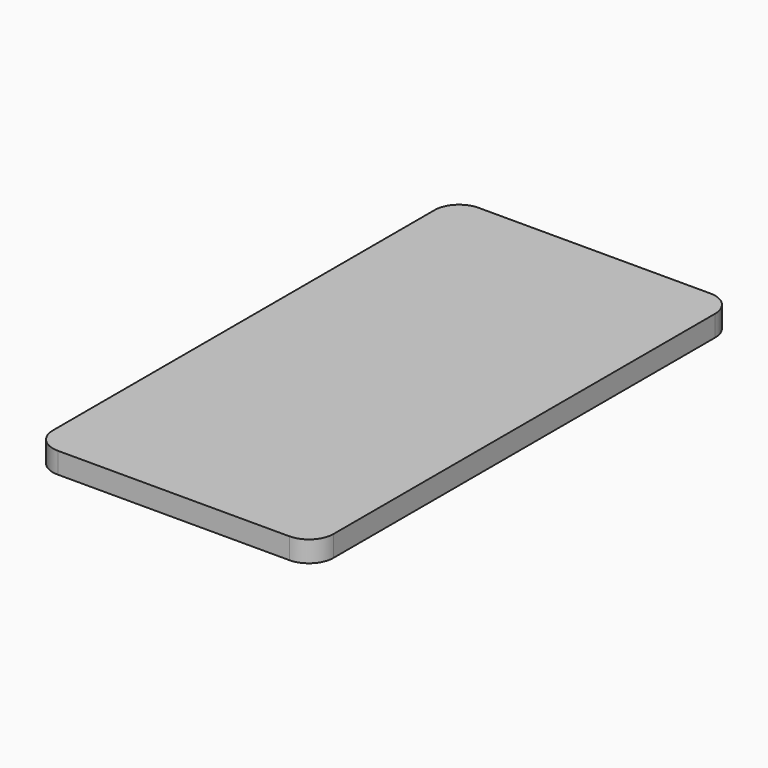
from build123d import *

# Parameters (mm, degrees)
F0_TEXT_SIZE = 202.7059043581
F1_DEPTH     = 152.4
F2_R         = 43.5227402162
F2_R_2       = 31.6103
F2_R_3       = 31.3528753957
F2_R_4       = 28.9308805731
F3_DEPTH     = 152.4
F5_DEPTH     = 154.4


# Not quite as in the source:
# - a feature names something its author has since deleted; it is built from what else it names
# - Text() gives the source's letters only with a copy of the font that has no kerning and outlines rounded to 1/6400 em; it was checked with that copy


with BuildPart() as f1:
    # F0 (on Top) → F1 (new body)
    with BuildSketch(Plane.XY):
        with BuildLine():
            ThreePointArc((0, -177.8), (-52.076414305, -52.076414305), (-177.8, 0))
            Line((-177.8, 0), (-1854.2, 0))
            ThreePointArc((-1854.2, 0), (-1979.923585695, -52.076414305), (-2032, -177.8))
            Line((-2032, -177.8), (-2032, -3632.2))
            ThreePointArc((-2032, -3632.2), (-1979.923585695, -3757.923585695), (-1854.2, -3810))
            Line((-1854.2, -3810), (-177.8, -3810))
            ThreePointArc((-177.8, -3810), (-52.076414305, -3757.923585695), (0, -3632.2))
            Line((0, -3632.2), (0, -177.8))
        make_face()
        with BuildLine():
            add(Edge.make_bspline(
                [(-1427.8888958164, -1437.0154963626), (-1420.3666063969, -1446.754881611), (-1420.3666063969, -1460.9126221185)],
                knots=[0, 0, 0, 1, 1, 1], degree=2))
            add(Edge.make_bspline(
                [(-1420.3666063969, -1460.9126221185), (-1420.3666063969, -1480.5180838057), (-1434.4768377081, -1491.8094361344)],
                knots=[0, 0, 0, 1, 1, 1], degree=2))
            add(Edge.make_bspline(
                [(-1434.4768377081, -1491.8094361344), (-1448.5870690193, -1503.1007884631), (-1473.7035974811, -1503.1007884631)],
                knots=[0, 0, 0, 1, 1, 1], degree=2))
            add(Edge.make_bspline(
                [(-1473.7035974811, -1503.1007884631), (-1496.8880852921, -1503.1007884631), (-1514.6881975185, -1494.3590963376)],
                knots=[0, 0, 0, 1, 1, 1], degree=2))
            Line((-1514.6881975185, -1494.3590963376), (-1514.6881975185, -1465.8535785372))
            add(Edge.make_bspline(
                [(-1514.6881975185, -1465.8535785372), (-1500.0553650477, -1472.4098476313), (-1489.904233431, -1475.070362626)],
                knots=[0, 0, 0, 1, 1, 1], degree=2))
            add(Edge.make_bspline(
                [(-1489.904233431, -1475.070362626), (-1479.7531018143, -1477.7308776207), (-1471.3281376644, -1477.7308776207)],
                knots=[0, 0, 0, 1, 1, 1], degree=2))
            add(Edge.make_bspline(
                [(-1471.3281376644, -1477.7308776207), (-1461.2561880416, -1477.7308776207), (-1455.8559760584, -1473.8826327177)],
                knots=[0, 0, 0, 1, 1, 1], degree=2))
            add(Edge.make_bspline(
                [(-1455.8559760584, -1473.8826327177), (-1450.4557640751, -1470.0343878146), (-1450.4557640751, -1462.4012436037)],
                knots=[0, 0, 0, 1, 1, 1], degree=2))
            add(Edge.make_bspline(
                [(-1450.4557640751, -1462.4012436037), (-1450.4557640751, -1458.1570887312), (-1452.8312238918, -1454.8314449878)],
                knots=[0, 0, 0, 1, 1, 1], degree=2))
            add(Edge.make_bspline(
                [(-1452.8312238918, -1454.8314449878), (-1455.2066837085, -1451.5058012444), (-1459.8150757529, -1448.4493762803)],
                knots=[0, 0, 0, 1, 1, 1], degree=2))
            add(Edge.make_bspline(
                [(-1459.8150757529, -1448.4493762803), (-1464.4234677972, -1445.3929513161), (-1478.5812083048, -1438.6466454367)],
                knots=[0, 0, 0, 1, 1, 1], degree=2))
            add(Edge.make_bspline(
                [(-1478.5812083048, -1438.6466454367), (-1491.8204376831, -1432.4071043182), (-1498.4558887711, -1426.6743279605)],
                knots=[0, 0, 0, 1, 1, 1], degree=2))
            add(Edge.make_bspline(
                [(-1498.4558887711, -1426.6743279605), (-1505.0913398591, -1420.9415516029), (-1509.0504395536, -1413.3084073919)],
                knots=[0, 0, 0, 1, 1, 1], degree=2))
            add(Edge.make_bspline(
                [(-1509.0504395536, -1413.3084073919), (-1513.0095392481, -1405.6752631809), (-1513.0095392481, -1395.5082951655)],
                knots=[0, 0, 0, 1, 1, 1], degree=2))
            add(Edge.make_bspline(
                [(-1513.0095392481, -1395.5082951655), (-1513.0095392481, -1376.282907049), (-1499.9920194526, -1365.3082826959)],
                knots=[0, 0, 0, 1, 1, 1], degree=2))
            add(Edge.make_bspline(
                [(-1499.9920194526, -1365.3082826959), (-1486.9744996571, -1354.3336583427), (-1464.011721429, -1354.3336583427)],
                knots=[0, 0, 0, 1, 1, 1], degree=2))
            add(Edge.make_bspline(
                [(-1464.011721429, -1354.3336583427), (-1452.7362054991, -1354.3336583427), (-1442.4900554897, -1356.9941733374)],
                knots=[0, 0, 0, 1, 1, 1], degree=2))
            add(Edge.make_bspline(
                [(-1442.4900554897, -1356.9941733374), (-1432.2439054804, -1359.6546883321), (-1421.0634079431, -1364.5006263582)],
                knots=[0, 0, 0, 1, 1, 1], degree=2))
            Line((-1421.0634079431, -1364.5006263582), (-1430.9453207806, -1388.3819157154))
            add(Edge.make_bspline(
                [(-1430.9453207806, -1388.3819157154), (-1442.5375646861, -1383.630996082), (-1450.107363302, -1381.7464646274)],
                knots=[0, 0, 0, 1, 1, 1], degree=2))
            add(Edge.make_bspline(
                [(-1450.107363302, -1381.7464646274), (-1457.6771619178, -1379.8619331728), (-1464.9935781533, -1379.8619331728)],
                knots=[0, 0, 0, 1, 1, 1], degree=2))
            add(Edge.make_bspline(
                [(-1464.9935781533, -1379.8619331728), (-1473.7035974811, -1379.8619331728), (-1478.3594987219, -1383.91605126)],
                knots=[0, 0, 0, 1, 1, 1], degree=2))
            add(Edge.make_bspline(
                [(-1478.3594987219, -1383.91605126), (-1483.0153999626, -1387.9701693472), (-1483.0153999626, -1394.4947656437)],
                knots=[0, 0, 0, 1, 1, 1], degree=2))
            add(Edge.make_bspline(
                [(-1483.0153999626, -1394.4947656437), (-1483.0153999626, -1398.5488837308), (-1481.130868508, -1401.5736358974)],
                knots=[0, 0, 0, 1, 1, 1], degree=2))
            add(Edge.make_bspline(
                [(-1481.130868508, -1401.5736358974), (-1479.2463370534, -1404.598388064), (-1475.1447097699, -1407.4172670465)],
                knots=[0, 0, 0, 1, 1, 1], degree=2))
            add(Edge.make_bspline(
                [(-1475.1447097699, -1407.4172670465), (-1471.0430824864, -1410.236146029), (-1455.7134484694, -1417.5525622644)],
                knots=[0, 0, 0, 1, 1, 1], degree=2))
            add(Edge.make_bspline(
                [(-1455.7134484694, -1417.5525622644), (-1435.411185236, -1427.2761111141), (-1427.8888958164, -1437.0154963626)],
                knots=[0, 0, 0, 1, 1, 1], degree=2))
        make_face(mode=Mode.SUBTRACT)
        Polygon((-1272.4863146081, -1501.105402217), (-1305.5527152566, -1501.105402217), (-1316.0364112476, -1466.6453984761), (-1368.8032919758, -1466.6453984761), (-1379.2869879668, -1501.105402217), (-1412.3533886153, -1501.105402217), (-1361.2651661575, -1355.7906070303), (-1323.7645738512, -1355.7906070303), align=None, mode=Mode.SUBTRACT)
        with BuildLine():
            Line((-1164.8938213106, -1501.105402217), (-1193.0192655402, -1501.105402217))
            Line((-1193.0192655402, -1501.105402217), (-1227.8593428518, -1387.5900957765))
            Line((-1227.8593428518, -1387.5900957765), (-1228.7461811834, -1387.5900957765))
            add(Edge.make_bspline(
                [(-1228.7461811834, -1387.5900957765), (-1226.84581333, -1422.2084635051), (-1226.84581333, -1433.8007074106)],
                knots=[0, 0, 0, 1, 1, 1], degree=2))
            Line((-1226.84581333, -1433.8007074106), (-1226.84581333, -1501.105402217))
            Line((-1226.84581333, -1501.105402217), (-1254.2744560135, -1501.105402217))
            Line((-1254.2744560135, -1501.105402217), (-1254.2744560135, -1356.3923901839))
            Line((-1254.2744560135, -1356.3923901839), (-1212.4980360372, -1356.3923901839))
            Line((-1212.4980360372, -1356.3923901839), (-1178.2597418792, -1467.0571448444))
            Line((-1178.2597418792, -1467.0571448444), (-1177.6579587256, -1467.0571448444))
            Line((-1177.6579587256, -1467.0571448444), (-1141.3292599289, -1356.3923901839))
            Line((-1141.3292599289, -1356.3923901839), (-1099.5845127502, -1356.3923901839))
            Line((-1099.5845127502, -1356.3923901839), (-1099.5845127502, -1501.105402217))
            Line((-1099.5845127502, -1501.105402217), (-1128.1850489432, -1501.105402217))
            Line((-1128.1850489432, -1501.105402217), (-1128.1850489432, -1432.5971411035))
            add(Edge.make_bspline(
                [(-1128.1850489432, -1432.5971411035), (-1128.1850489432, -1427.7512030774), (-1128.0266849554, -1421.4166435662)],
                knots=[0, 0, 0, 1, 1, 1], degree=2))
            add(Edge.make_bspline(
                [(-1128.0266849554, -1421.4166435662), (-1127.8683209676, -1415.082084055), (-1126.6964274581, -1387.7801325618)],
                knots=[0, 0, 0, 1, 1, 1], degree=2))
            Line((-1126.6964274581, -1387.7801325618), (-1127.5832657896, -1387.7801325618))
            Line((-1127.5832657896, -1387.7801325618), (-1164.8938213106, -1501.105402217))
        make_face(mode=Mode.SUBTRACT)
        with BuildLine():
            add(Edge.make_bspline(
                [(-985.2615499719, -1437.0154963626), (-977.7392605524, -1446.754881611), (-977.7392605524, -1460.9126221185)],
                knots=[0, 0, 0, 1, 1, 1], degree=2))
            add(Edge.make_bspline(
                [(-977.7392605524, -1460.9126221185), (-977.7392605524, -1480.5180838057), (-991.8494918636, -1491.8094361344)],
                knots=[0, 0, 0, 1, 1, 1], degree=2))
            add(Edge.make_bspline(
                [(-991.8494918636, -1491.8094361344), (-1005.9597231748, -1503.1007884631), (-1031.0762516366, -1503.1007884631)],
                knots=[0, 0, 0, 1, 1, 1], degree=2))
            add(Edge.make_bspline(
                [(-1031.0762516366, -1503.1007884631), (-1054.2607394476, -1503.1007884631), (-1072.060851674, -1494.3590963376)],
                knots=[0, 0, 0, 1, 1, 1], degree=2))
            Line((-1072.060851674, -1494.3590963376), (-1072.060851674, -1465.8535785372))
            add(Edge.make_bspline(
                [(-1072.060851674, -1465.8535785372), (-1057.4280192032, -1472.4098476313), (-1047.2768875865, -1475.070362626)],
                knots=[0, 0, 0, 1, 1, 1], degree=2))
            add(Edge.make_bspline(
                [(-1047.2768875865, -1475.070362626), (-1037.1257559698, -1477.7308776207), (-1028.7007918199, -1477.7308776207)],
                knots=[0, 0, 0, 1, 1, 1], degree=2))
            add(Edge.make_bspline(
                [(-1028.7007918199, -1477.7308776207), (-1018.6288421971, -1477.7308776207), (-1013.2286302139, -1473.8826327177)],
                knots=[0, 0, 0, 1, 1, 1], degree=2))
            add(Edge.make_bspline(
                [(-1013.2286302139, -1473.8826327177), (-1007.8284182306, -1470.0343878146), (-1007.8284182306, -1462.4012436037)],
                knots=[0, 0, 0, 1, 1, 1], degree=2))
            add(Edge.make_bspline(
                [(-1007.8284182306, -1462.4012436037), (-1007.8284182306, -1458.1570887312), (-1010.2038780473, -1454.8314449878)],
                knots=[0, 0, 0, 1, 1, 1], degree=2))
            add(Edge.make_bspline(
                [(-1010.2038780473, -1454.8314449878), (-1012.579337864, -1451.5058012444), (-1017.1877299083, -1448.4493762803)],
                knots=[0, 0, 0, 1, 1, 1], degree=2))
            add(Edge.make_bspline(
                [(-1017.1877299083, -1448.4493762803), (-1021.7961219527, -1445.3929513161), (-1035.9538624603, -1438.6466454367)],
                knots=[0, 0, 0, 1, 1, 1], degree=2))
            add(Edge.make_bspline(
                [(-1035.9538624603, -1438.6466454367), (-1049.1930918386, -1432.4071043182), (-1055.8285429266, -1426.6743279605)],
                knots=[0, 0, 0, 1, 1, 1], degree=2))
            add(Edge.make_bspline(
                [(-1055.8285429266, -1426.6743279605), (-1062.4639940146, -1420.9415516029), (-1066.4230937091, -1413.3084073919)],
                knots=[0, 0, 0, 1, 1, 1], degree=2))
            add(Edge.make_bspline(
                [(-1066.4230937091, -1413.3084073919), (-1070.3821934036, -1405.6752631809), (-1070.3821934036, -1395.5082951655)],
                knots=[0, 0, 0, 1, 1, 1], degree=2))
            add(Edge.make_bspline(
                [(-1070.3821934036, -1395.5082951655), (-1070.3821934036, -1376.282907049), (-1057.3646736081, -1365.3082826959)],
                knots=[0, 0, 0, 1, 1, 1], degree=2))
            add(Edge.make_bspline(
                [(-1057.3646736081, -1365.3082826959), (-1044.3471538126, -1354.3336583427), (-1021.3843755845, -1354.3336583427)],
                knots=[0, 0, 0, 1, 1, 1], degree=2))
            add(Edge.make_bspline(
                [(-1021.3843755845, -1354.3336583427), (-1010.1088596546, -1354.3336583427), (-999.8627096452, -1356.9941733374)],
                knots=[0, 0, 0, 1, 1, 1], degree=2))
            add(Edge.make_bspline(
                [(-999.8627096452, -1356.9941733374), (-989.6165596359, -1359.6546883321), (-978.4360620986, -1364.5006263582)],
                knots=[0, 0, 0, 1, 1, 1], degree=2))
            Line((-978.4360620986, -1364.5006263582), (-988.3179749361, -1388.3819157154))
            add(Edge.make_bspline(
                [(-988.3179749361, -1388.3819157154), (-999.9102188416, -1383.630996082), (-1007.4800174574, -1381.7464646274)],
                knots=[0, 0, 0, 1, 1, 1], degree=2))
            add(Edge.make_bspline(
                [(-1007.4800174574, -1381.7464646274), (-1015.0498160733, -1379.8619331728), (-1022.3662323087, -1379.8619331728)],
                knots=[0, 0, 0, 1, 1, 1], degree=2))
            add(Edge.make_bspline(
                [(-1022.3662323087, -1379.8619331728), (-1031.0762516366, -1379.8619331728), (-1035.7321528774, -1383.91605126)],
                knots=[0, 0, 0, 1, 1, 1], degree=2))
            add(Edge.make_bspline(
                [(-1035.7321528774, -1383.91605126), (-1040.3880541181, -1387.9701693472), (-1040.3880541181, -1394.4947656437)],
                knots=[0, 0, 0, 1, 1, 1], degree=2))
            add(Edge.make_bspline(
                [(-1040.3880541181, -1394.4947656437), (-1040.3880541181, -1398.5488837308), (-1038.5035226635, -1401.5736358974)],
                knots=[0, 0, 0, 1, 1, 1], degree=2))
            add(Edge.make_bspline(
                [(-1038.5035226635, -1401.5736358974), (-1036.6189912089, -1404.598388064), (-1032.5173639254, -1407.4172670465)],
                knots=[0, 0, 0, 1, 1, 1], degree=2))
            add(Edge.make_bspline(
                [(-1032.5173639254, -1407.4172670465), (-1028.4157366419, -1410.236146029), (-1013.0861026249, -1417.5525622644)],
                knots=[0, 0, 0, 1, 1, 1], degree=2))
            add(Edge.make_bspline(
                [(-1013.0861026249, -1417.5525622644), (-992.7838393915, -1427.2761111141), (-985.2615499719, -1437.0154963626)],
                knots=[0, 0, 0, 1, 1, 1], degree=2))
        make_face(mode=Mode.SUBTRACT)
        with BuildLine():
            Line((-864.3189725045, -1356.3923901839), (-833.7230500655, -1356.3923901839))
            Line((-833.7230500655, -1356.3923901839), (-833.7230500655, -1450.0171797593))
            add(Edge.make_bspline(
                [(-833.7230500655, -1450.0171797593), (-833.7230500655, -1466.0752881201), (-840.8969387119, -1478.142623989)],
                knots=[0, 0, 0, 1, 1, 1], degree=2))
            add(Edge.make_bspline(
                [(-840.8969387119, -1478.142623989), (-848.0708273583, -1490.2099598578), (-861.642621111, -1496.6553741604)],
                knots=[0, 0, 0, 1, 1, 1], degree=2))
            add(Edge.make_bspline(
                [(-861.642621111, -1496.6553741604), (-875.2144148638, -1503.1007884631), (-893.7113286364, -1503.1007884631)],
                knots=[0, 0, 0, 1, 1, 1], degree=2))
            add(Edge.make_bspline(
                [(-893.7113286364, -1503.1007884631), (-921.6150632832, -1503.1007884631), (-937.0555520918, -1488.7846839678)],
                knots=[0, 0, 0, 1, 1, 1], degree=2))
            add(Edge.make_bspline(
                [(-937.0555520918, -1488.7846839678), (-952.4960409003, -1474.4685794725), (-952.4960409003, -1449.6371061886)],
                knots=[0, 0, 0, 1, 1, 1], degree=2))
            Line((-952.4960409003, -1449.6371061886), (-952.4960409003, -1356.3923901839))
            Line((-952.4960409003, -1356.3923901839), (-921.9317912588, -1356.3923901839))
            Line((-921.9317912588, -1356.3923901839), (-921.9317912588, -1444.9812049479))
            add(Edge.make_bspline(
                [(-921.9317912588, -1444.9812049479), (-921.9317912588, -1461.7044420574), (-915.2013217782, -1469.5276230537)],
                knots=[0, 0, 0, 1, 1, 1], degree=2))
            add(Edge.make_bspline(
                [(-915.2013217782, -1469.5276230537), (-908.4708522975, -1477.3508040501), (-892.9195086976, -1477.3508040501)],
                knots=[0, 0, 0, 1, 1, 1], degree=2))
            add(Edge.make_bspline(
                [(-892.9195086976, -1477.3508040501), (-877.8749298585, -1477.3508040501), (-871.0969511815, -1469.4801138574)],
                knots=[0, 0, 0, 1, 1, 1], degree=2))
            add(Edge.make_bspline(
                [(-871.0969511815, -1469.4801138574), (-864.3189725045, -1461.6094236648), (-864.3189725045, -1444.7911681625)],
                knots=[0, 0, 0, 1, 1, 1], degree=2))
            Line((-864.3189725045, -1444.7911681625), (-864.3189725045, -1356.3923901839))
        make_face(mode=Mode.SUBTRACT)
        with BuildLine():
            Line((-669.9113411061, -1356.3923901839), (-669.9113411061, -1501.105402217))
            Line((-669.9113411061, -1501.105402217), (-708.9005548974, -1501.105402217))
            Line((-708.9005548974, -1501.105402217), (-771.8660764387, -1391.6442138636))
            Line((-771.8660764387, -1391.6442138636), (-772.7529147702, -1391.6442138636))
            add(Edge.make_bspline(
                [(-772.7529147702, -1391.6442138636), (-770.8525469169, -1420.6248236273), (-770.8525469169, -1433.0088874717)],
                knots=[0, 0, 0, 1, 1, 1], degree=2))
            Line((-770.8525469169, -1433.0088874717), (-770.8525469169, -1501.105402217))
            Line((-770.8525469169, -1501.105402217), (-798.2811896003, -1501.105402217))
            Line((-798.2811896003, -1501.105402217), (-798.2811896003, -1356.3923901839))
            Line((-798.2811896003, -1356.3923901839), (-759.577030987, -1356.3923901839))
            Line((-759.577030987, -1356.3923901839), (-696.738200636, -1464.7767034203))
            Line((-696.738200636, -1464.7767034203), (-696.0413990897, -1464.7767034203))
            add(Edge.make_bspline(
                [(-696.0413990897, -1464.7767034203), (-697.5300205748, -1436.556240798), (-697.5300205748, -1424.9006512974)],
                knots=[0, 0, 0, 1, 1, 1], degree=2))
            Line((-697.5300205748, -1424.9006512974), (-697.5300205748, -1356.3923901839))
            Line((-697.5300205748, -1356.3923901839), (-669.9113411061, -1356.3923901839))
        make_face(mode=Mode.SUBTRACT)
        with BuildLine():
            Line((-578.5669929547, -1445.3929513161), (-578.5669929547, -1419.8330036884))
            Line((-578.5669929547, -1419.8330036884), (-521.1442109857, -1419.8330036884))
            Line((-521.1442109857, -1419.8330036884), (-521.1442109857, -1494.8658610985))
            add(Edge.make_bspline(
                [(-521.1442109857, -1494.8658610985), (-535.1119147079, -1499.4267439466), (-547.4326329572, -1501.2637662048)],
                knots=[0, 0, 0, 1, 1, 1], degree=2))
            add(Edge.make_bspline(
                [(-547.4326329572, -1501.2637662048), (-559.7533512064, -1503.1007884631), (-572.6125070142, -1503.1007884631)],
                knots=[0, 0, 0, 1, 1, 1], degree=2))
            add(Edge.make_bspline(
                [(-572.6125070142, -1503.1007884631), (-605.362179687, -1503.1007884631), (-622.6396907538, -1483.843727549)],
                knots=[0, 0, 0, 1, 1, 1], degree=2))
            add(Edge.make_bspline(
                [(-622.6396907538, -1483.843727549), (-639.9172018206, -1464.586666635), (-639.9172018206, -1428.5430230163)],
                knots=[0, 0, 0, 1, 1, 1], degree=2))
            add(Edge.make_bspline(
                [(-639.9172018206, -1428.5430230163), (-639.9172018206, -1393.5129089194), (-619.8683209676, -1373.9232836311)],
                knots=[0, 0, 0, 1, 1, 1], degree=2))
            add(Edge.make_bspline(
                [(-619.8683209676, -1373.9232836311), (-599.8194401147, -1354.3336583427), (-564.3142340545, -1354.3336583427)],
                knots=[0, 0, 0, 1, 1, 1], degree=2))
            add(Edge.make_bspline(
                [(-564.3142340545, -1354.3336583427), (-542.0165845751, -1354.3336583427), (-521.3342477711, -1363.2337144559)],
                knots=[0, 0, 0, 1, 1, 1], degree=2))
            Line((-521.3342477711, -1363.2337144559), (-531.5328885841, -1387.7801325618))
            add(Edge.make_bspline(
                [(-531.5328885841, -1387.7801325618), (-547.3692873621, -1379.8619331728), (-564.5042708398, -1379.8619331728)],
                knots=[0, 0, 0, 1, 1, 1], degree=2))
            add(Edge.make_bspline(
                [(-564.5042708398, -1379.8619331728), (-584.394787705, -1379.8619331728), (-596.3671051811, -1393.2278537414)],
                knots=[0, 0, 0, 1, 1, 1], degree=2))
            add(Edge.make_bspline(
                [(-596.3671051811, -1393.2278537414), (-608.3394226573, -1406.5937743101), (-608.3394226573, -1429.1448061699)],
                knots=[0, 0, 0, 1, 1, 1], degree=2))
            add(Edge.make_bspline(
                [(-608.3394226573, -1429.1448061699), (-608.3394226573, -1452.7093675515), (-598.6950558015, -1465.1251041935)],
                knots=[0, 0, 0, 1, 1, 1], degree=2))
            add(Edge.make_bspline(
                [(-598.6950558015, -1465.1251041935), (-589.0506889457, -1477.5408408354), (-570.6487935657, -1477.5408408354)],
                knots=[0, 0, 0, 1, 1, 1], degree=2))
            add(Edge.make_bspline(
                [(-570.6487935657, -1477.5408408354), (-561.0202631087, -1477.5408408354), (-551.1383502712, -1475.5771273869)],
                knots=[0, 0, 0, 1, 1, 1], degree=2))
            Line((-551.1383502712, -1475.5771273869), (-551.1383502712, -1445.3929513161))
            Line((-551.1383502712, -1445.3929513161), (-578.5669929547, -1445.3929513161))
        make_face(mode=Mode.SUBTRACT)
        with BuildLine():
            ThreePointArc((-1206.5, -567.7571510792), (-1176.7420489686, -495.9151021106), (-1104.9, -466.1571510792))
            Line((-1104.9, -466.1571510792), (-927.1, -466.1571510792))
            ThreePointArc((-927.1, -466.1571510792), (-855.2579510314, -495.9151021106), (-825.5, -567.7571510792))
            Line((-825.5, -567.7571510792), (-825.5, -745.5571510792))
            ThreePointArc((-825.5, -745.5571510792), (-855.2579510314, -817.3992000477), (-927.1, -847.1571510792))
            Line((-927.1, -847.1571510792), (-1104.9, -847.1571510792))
            ThreePointArc((-1104.9, -847.1571510792), (-1176.7420489686, -817.3992000477), (-1206.5, -745.5571510792))
            Line((-1206.5, -745.5571510792), (-1206.5, -567.7571510792))
        make_face(mode=Mode.SUBTRACT)
        with BuildLine():
            Line((-647.7, -796.3571510792), (-647.7, -516.9571510792))
            ThreePointArc((-647.7, -516.9571510792), (-632.8210244843, -481.0361265949), (-596.9, -466.1571510792))
            Line((-596.9, -466.1571510792), (-571.5, -466.1571510792))
            ThreePointArc((-571.5, -466.1571510792), (-535.5789755157, -481.0361265949), (-520.7, -516.9571510792))
            Line((-520.7, -516.9571510792), (-520.7, -796.3571510792))
            ThreePointArc((-520.7, -796.3571510792), (-535.5789755157, -832.2781755635), (-571.5, -847.1571510792))
            Line((-571.5, -847.1571510792), (-596.9, -847.1571510792))
            ThreePointArc((-596.9, -847.1571510792), (-632.8210244843, -832.2781755635), (-647.7, -796.3571510792))
        make_face(mode=Mode.SUBTRACT)
        with BuildLine():
            Line((-927.1, -466.1571510792), (-1104.9, -466.1571510792))
            ThreePointArc((-1104.9, -466.1571510792), (-1176.7420489686, -495.9151021106), (-1206.5, -567.7571510792))
            Line((-1206.5, -567.7571510792), (-1206.5, -745.5571510792))
            ThreePointArc((-1206.5, -745.5571510792), (-1176.7420489686, -817.3992000477), (-1104.9, -847.1571510792))
            Line((-1104.9, -847.1571510792), (-927.1, -847.1571510792))
            ThreePointArc((-927.1, -847.1571510792), (-855.2579510314, -817.3992000477), (-825.5, -745.5571510792))
            Line((-825.5, -745.5571510792), (-825.5, -567.7571510792))
            ThreePointArc((-825.5, -567.7571510792), (-855.2579510314, -495.9151021106), (-927.1, -466.1571510792))
        make_face()
        with BuildLine():
            ThreePointArc((-1181.1, -567.7571510792), (-1158.7815367264, -513.8756143528), (-1104.9, -491.5571510792))
            Line((-1104.9, -491.5571510792), (-927.1, -491.5571510792))
            ThreePointArc((-927.1, -491.5571510792), (-873.2184632736, -513.8756143528), (-850.9, -567.7571510792))
            Line((-850.9, -567.7571510792), (-850.9, -745.5571510792))
            ThreePointArc((-850.9, -745.5571510792), (-873.2184632736, -799.4386878056), (-927.1, -821.7571510792))
            Line((-927.1, -821.7571510792), (-1104.9, -821.7571510792))
            ThreePointArc((-1104.9, -821.7571510792), (-1158.7815367264, -799.4386878056), (-1181.1, -745.5571510792))
            Line((-1181.1, -745.5571510792), (-1181.1, -567.7571510792))
        make_face(mode=Mode.SUBTRACT)
        with BuildLine():
            Line((-927.1, -491.5571510792), (-1104.9, -491.5571510792))
            ThreePointArc((-1104.9, -491.5571510792), (-1158.7815367264, -513.8756143528), (-1181.1, -567.7571510792))
            Line((-1181.1, -567.7571510792), (-1181.1, -745.5571510792))
            ThreePointArc((-1181.1, -745.5571510792), (-1158.7815367264, -799.4386878056), (-1104.9, -821.7571510792))
            Line((-1104.9, -821.7571510792), (-927.1, -821.7571510792))
            ThreePointArc((-927.1, -821.7571510792), (-873.2184632736, -799.4386878056), (-850.9, -745.5571510792))
            Line((-850.9, -745.5571510792), (-850.9, -567.7571510792))
            ThreePointArc((-850.9, -567.7571510792), (-873.2184632736, -513.8756143528), (-927.1, -491.5571510792))
        make_face()
        with BuildLine():
            ThreePointArc((-596.9, -466.1571510792), (-632.8210244843, -481.0361265949), (-647.7, -516.9571510792))
            Line((-647.7, -516.9571510792), (-647.7, -796.3571510792))
            ThreePointArc((-647.7, -796.3571510792), (-632.8210244843, -832.2781755635), (-596.9, -847.1571510792))
            Line((-596.9, -847.1571510792), (-571.5, -847.1571510792))
            ThreePointArc((-571.5, -847.1571510792), (-535.5789755157, -832.2781755635), (-520.7, -796.3571510792))
            Line((-520.7, -796.3571510792), (-520.7, -516.9571510792))
            ThreePointArc((-520.7, -516.9571510792), (-535.5789755157, -481.0361265949), (-571.5, -466.1571510792))
            Line((-571.5, -466.1571510792), (-596.9, -466.1571510792))
        make_face()
        with BuildLine():
            ThreePointArc((-635, -516.9571510792), (-623.8407683632, -490.016382716), (-596.9, -478.8571510792))
            Line((-596.9, -478.8571510792), (-571.5, -478.8571510792))
            ThreePointArc((-571.5, -478.8571510792), (-544.5592316368, -490.016382716), (-533.4, -516.9571510792))
            Line((-533.4, -516.9571510792), (-533.4, -796.3571510792))
            ThreePointArc((-533.4, -796.3571510792), (-544.5592316368, -823.2979194424), (-571.5, -834.4571510792))
            Line((-571.5, -834.4571510792), (-596.9, -834.4571510792))
            ThreePointArc((-596.9, -834.4571510792), (-623.8407683632, -823.2979194424), (-635, -796.3571510792))
            Line((-635, -796.3571510792), (-635, -516.9571510792))
        make_face(mode=Mode.SUBTRACT)
        with BuildLine():
            Line((-571.5, -478.8571510792), (-596.9, -478.8571510792))
            ThreePointArc((-596.9, -478.8571510792), (-623.8407683632, -490.016382716), (-635, -516.9571510792))
            Line((-635, -516.9571510792), (-635, -796.3571510792))
            ThreePointArc((-635, -796.3571510792), (-623.8407683632, -823.2979194424), (-596.9, -834.4571510792))
            Line((-596.9, -834.4571510792), (-571.5, -834.4571510792))
            ThreePointArc((-571.5, -834.4571510792), (-544.5592316368, -823.2979194424), (-533.4, -796.3571510792))
            Line((-533.4, -796.3571510792), (-533.4, -516.9571510792))
            ThreePointArc((-533.4, -516.9571510792), (-544.5592316368, -490.016382716), (-571.5, -478.8571510792))
        make_face()
        with BuildLine():
            ThreePointArc((-596.9, -821.247279644), (-614.4999786928, -813.957129772), (-621.7901285648, -796.3571510792))
            Line((-621.7901285648, -796.3571510792), (-621.7901285648, -629.9103599742))
            ThreePointArc((-621.7901285648, -629.9103599742), (-614.9559919258, -613.4112946132), (-598.4569265648, -606.5771579742))
            Line((-598.4569265648, -606.5771579742), (-569.9430734352, -606.5771579742))
            ThreePointArc((-569.9430734352, -606.5771579742), (-553.4440080742, -613.4112946132), (-546.6098714352, -629.9103599742))
            Line((-546.6098714352, -629.9103599742), (-546.6098714352, -796.3571510792))
            ThreePointArc((-546.6098714352, -796.3571510792), (-553.9000213072, -813.957129772), (-571.5, -821.247279644))
            Line((-571.5, -821.247279644), (-596.9, -821.247279644))
        make_face(mode=Mode.SUBTRACT)
        with BuildLine():
            ThreePointArc((-571.5, -493.6239421368), (-555.00092973, -500.4580808092), (-548.1667910576, -516.9571510792))
            Line((-548.1667910576, -516.9571510792), (-548.1667910576, -546.4907401368))
            ThreePointArc((-548.1667910576, -546.4907401368), (-555.0009276966, -562.9898054978), (-571.4999930576, -569.8239421368))
            Line((-571.4999930576, -569.8239421368), (-584.2, -569.8239421368))
            Line((-584.2, -569.8239421368), (-596.9000069424, -569.8239421368))
            ThreePointArc((-596.9000069424, -569.8239421368), (-613.3990723034, -562.9898054978), (-620.2332089424, -546.4907401368))
            Line((-620.2332089424, -546.4907401368), (-620.2332089424, -516.9571510792))
            ThreePointArc((-620.2332089424, -516.9571510792), (-613.39907027, -500.4580808092), (-596.9, -493.6239421368))
            Line((-596.9, -493.6239421368), (-571.5, -493.6239421368))
        make_face(mode=Mode.SUBTRACT)
        with BuildLine():
            Line((-621.7901285648, -629.9103599742), (-621.7901285648, -796.3571510792))
            ThreePointArc((-621.7901285648, -796.3571510792), (-614.4999786928, -813.957129772), (-596.9, -821.247279644))
            Line((-596.9, -821.247279644), (-571.5, -821.247279644))
            ThreePointArc((-571.5, -821.247279644), (-553.9000213072, -813.957129772), (-546.6098714352, -796.3571510792))
            Line((-546.6098714352, -796.3571510792), (-546.6098714352, -629.9103599742))
            ThreePointArc((-546.6098714352, -629.9103599742), (-553.4440080742, -613.4112946132), (-569.9430734352, -606.5771579742))
            Line((-569.9430734352, -606.5771579742), (-598.4569265648, -606.5771579742))
            ThreePointArc((-598.4569265648, -606.5771579742), (-614.9559919258, -613.4112946132), (-621.7901285648, -629.9103599742))
        make_face()
        with Locations((-1524, -1501.105402217)):
            Text('SAMSUNG', F0_TEXT_SIZE, font='Open Sans', font_style=FontStyle.BOLD, text_align=(TextAlign.LEFT, TextAlign.BOTTOM))
        with BuildLine():
            Line((-548.1667910576, -546.4907401368), (-548.1667910576, -516.9571510792))
            ThreePointArc((-548.1667910576, -516.9571510792), (-555.00092973, -500.4580808092), (-571.5, -493.6239421368))
            Line((-571.5, -493.6239421368), (-596.9, -493.6239421368))
            ThreePointArc((-596.9, -493.6239421368), (-613.39907027, -500.4580808092), (-620.2332089424, -516.9571510792))
            Line((-620.2332089424, -516.9571510792), (-620.2332089424, -546.4907401368))
            ThreePointArc((-620.2332089424, -546.4907401368), (-613.3990723034, -562.9898054978), (-596.9000069424, -569.8239421368))
            Line((-596.9000069424, -569.8239421368), (-584.2, -569.8239421368))
            Line((-584.2, -569.8239421368), (-571.4999930576, -569.8239421368))
            ThreePointArc((-571.4999930576, -569.8239421368), (-555.0009276966, -562.9898054978), (-548.1667910576, -546.4907401368))
        make_face()
        with BuildLine():
            Line((-1361.0751293722, -1440.9270868607), (-1323.3845002806, -1440.9270868607))
            add(Edge.make_bspline(
                [(-1323.3845002806, -1440.9270868607), (-1337.9223143588, -1394.114692073), (-1339.759336617, -1387.9701693472)],
                knots=[0, 0, 0, 1, 1, 1], degree=2))
            add(Edge.make_bspline(
                [(-1339.759336617, -1387.9701693472), (-1341.5963588752, -1381.8256466213), (-1342.3881788141, -1378.278293295)],
                knots=[0, 0, 0, 1, 1, 1], degree=2))
            add(Edge.make_bspline(
                [(-1342.3881788141, -1378.278293295), (-1345.6504769624, -1390.9474123174), (-1361.0751293722, -1440.9270868607)],
                knots=[0, 0, 0, 1, 1, 1], degree=2))
        make_face()
    extrude(amount=-F1_DEPTH)

    # F2 (on face) → F5 (join)
    with BuildSketch(Plane.XY):
        Polygon((-1143, -152.4), (-1016, -152.4), (-889, -152.4), (-889, -101.6), (-1016, -101.6), (-1143, -101.6), align=None)
        with Locations((-787.4, -127)):
            Circle(F2_R_2)
        with Locations((-711.2, -127)):
            Circle(F2_R_3)
        with Locations((-1397, -127)):
            Circle(F2_R)
        with Locations((-1397, -127)):
            Circle(F2_R_4, mode=Mode.SUBTRACT)
        with BuildLine():
            Line((-1168.4, -3719.4534733344), (-1016, -3719.4534733344))
            Line((-1016, -3719.4534733344), (-863.6, -3719.4534733344))
            ThreePointArc((-863.6, -3719.4534733344), (-836.6592316368, -3708.2942416976), (-825.5, -3681.3534733344))
            Line((-825.5, -3681.3534733344), (-825.5, -3630.5534733344))
            ThreePointArc((-825.5, -3630.5534733344), (-836.6592316368, -3603.6127049712), (-863.6, -3592.4534733344))
            Line((-863.6, -3592.4534733344), (-1016, -3592.4534733344))
            Line((-1016, -3592.4534733344), (-1168.4, -3592.4534733344))
            ThreePointArc((-1168.4, -3592.4534733344), (-1195.3407683632, -3603.6127049712), (-1206.5, -3630.5534733344))
            Line((-1206.5, -3630.5534733344), (-1206.5, -3681.3534733344))
            ThreePointArc((-1206.5, -3681.3534733344), (-1195.3407683632, -3708.2942416976), (-1168.4, -3719.4534733344))
        make_face()
    extrude(amount=-F5_DEPTH)


with BuildPart() as f3:
    # F2 (on face) → F3 (new body)
    with BuildSketch(Plane.XY):
        with BuildLine():
            Line((-177.8, 0), (-1016, 0))
            Line((-1016, 0), (-1854.2, 0))
            ThreePointArc((-1854.2, 0), (-1979.923585695, -52.076414305), (-2032, -177.8))
            Line((-2032, -177.8), (-2032, -3632.2))
            ThreePointArc((-2032, -3632.2), (-1979.923585695, -3757.923585695), (-1854.2, -3810))
            Line((-1854.2, -3810), (-177.8, -3810))
            ThreePointArc((-177.8, -3810), (-52.076414305, -3757.923585695), (0, -3632.2))
            Line((0, -3632.2), (0, -177.8))
            ThreePointArc((0, -177.8), (-52.076414305, -52.076414305), (-177.8, 0))
        make_face()
        with BuildLine():
            Line((-863.6, -3719.4534733344), (-1016, -3719.4534733344))
            Line((-1016, -3719.4534733344), (-1168.4, -3719.4534733344))
            ThreePointArc((-1168.4, -3719.4534733344), (-1195.3407683632, -3708.2942416976), (-1206.5, -3681.3534733344))
            Line((-1206.5, -3681.3534733344), (-1206.5, -3630.5534733344))
            ThreePointArc((-1206.5, -3630.5534733344), (-1195.3407683632, -3603.6127049712), (-1168.4, -3592.4534733344))
            Line((-1168.4, -3592.4534733344), (-1016, -3592.4534733344))
            Line((-1016, -3592.4534733344), (-863.6, -3592.4534733344))
            ThreePointArc((-863.6, -3592.4534733344), (-836.6592316368, -3603.6127049712), (-825.5, -3630.5534733344))
            Line((-825.5, -3630.5534733344), (-825.5, -3681.3534733344))
            ThreePointArc((-825.5, -3681.3534733344), (-836.6592316368, -3708.2942416976), (-863.6, -3719.4534733344))
        make_face(mode=Mode.SUBTRACT)
        Polygon((-25.4, -3516.2534733344), (-1016, -3516.2534733344), (-2006.6, -3516.2534733344), (-2006.6, -304.8), (-1016, -304.8), (-25.4, -304.8), align=None, mode=Mode.SUBTRACT)
        with Locations((-1397, -127)):
            Circle(F2_R, mode=Mode.SUBTRACT)
        Polygon((-889, -152.4), (-1016, -152.4), (-1143, -152.4), (-1143, -101.6), (-1016, -101.6), (-889, -101.6), align=None, mode=Mode.SUBTRACT)
        with Locations((-787.4, -127)):
            Circle(F2_R_2, mode=Mode.SUBTRACT)
        with Locations((-711.2, -127)):
            Circle(F2_R_3, mode=Mode.SUBTRACT)
        Polygon((-2006.6, -3516.2534733344), (-1016, -3516.2534733344), (-25.4, -3516.2534733344), (-25.4, -304.8), (-1016, -304.8), (-2006.6, -304.8), align=None)
        with BuildLine():
            add(Edge.make_bspline(
                [(-1455.7134484694, -1417.5525622644), (-1435.411185236, -1427.2761111141), (-1427.8888958164, -1437.0154963626)],
                knots=[0, 0, 0, 1, 1, 1], degree=2))
            add(Edge.make_bspline(
                [(-1427.8888958164, -1437.0154963626), (-1420.3666063969, -1446.754881611), (-1420.3666063969, -1460.9126221185)],
                knots=[0, 0, 0, 1, 1, 1], degree=2))
            add(Edge.make_bspline(
                [(-1420.3666063969, -1460.9126221185), (-1420.3666063969, -1480.5180838057), (-1434.4768377081, -1491.8094361344)],
                knots=[0, 0, 0, 1, 1, 1], degree=2))
            add(Edge.make_bspline(
                [(-1434.4768377081, -1491.8094361344), (-1448.5870690193, -1503.1007884631), (-1473.7035974811, -1503.1007884631)],
                knots=[0, 0, 0, 1, 1, 1], degree=2))
            add(Edge.make_bspline(
                [(-1473.7035974811, -1503.1007884631), (-1496.8880852921, -1503.1007884631), (-1514.6881975185, -1494.3590963376)],
                knots=[0, 0, 0, 1, 1, 1], degree=2))
            Line((-1514.6881975185, -1494.3590963376), (-1514.6881975185, -1465.8535785372))
            add(Edge.make_bspline(
                [(-1514.6881975185, -1465.8535785372), (-1500.0553650477, -1472.4098476313), (-1489.904233431, -1475.070362626)],
                knots=[0, 0, 0, 1, 1, 1], degree=2))
            add(Edge.make_bspline(
                [(-1489.904233431, -1475.070362626), (-1479.7531018143, -1477.7308776207), (-1471.3281376644, -1477.7308776207)],
                knots=[0, 0, 0, 1, 1, 1], degree=2))
            add(Edge.make_bspline(
                [(-1471.3281376644, -1477.7308776207), (-1461.2561880416, -1477.7308776207), (-1455.8559760584, -1473.8826327177)],
                knots=[0, 0, 0, 1, 1, 1], degree=2))
            add(Edge.make_bspline(
                [(-1455.8559760584, -1473.8826327177), (-1450.4557640751, -1470.0343878146), (-1450.4557640751, -1462.4012436037)],
                knots=[0, 0, 0, 1, 1, 1], degree=2))
            add(Edge.make_bspline(
                [(-1450.4557640751, -1462.4012436037), (-1450.4557640751, -1458.1570887312), (-1452.8312238918, -1454.8314449878)],
                knots=[0, 0, 0, 1, 1, 1], degree=2))
            add(Edge.make_bspline(
                [(-1452.8312238918, -1454.8314449878), (-1455.2066837085, -1451.5058012444), (-1459.8150757529, -1448.4493762803)],
                knots=[0, 0, 0, 1, 1, 1], degree=2))
            add(Edge.make_bspline(
                [(-1459.8150757529, -1448.4493762803), (-1464.4234677972, -1445.3929513161), (-1478.5812083048, -1438.6466454367)],
                knots=[0, 0, 0, 1, 1, 1], degree=2))
            add(Edge.make_bspline(
                [(-1478.5812083048, -1438.6466454367), (-1491.8204376831, -1432.4071043182), (-1498.4558887711, -1426.6743279605)],
                knots=[0, 0, 0, 1, 1, 1], degree=2))
            add(Edge.make_bspline(
                [(-1498.4558887711, -1426.6743279605), (-1505.0913398591, -1420.9415516029), (-1509.0504395536, -1413.3084073919)],
                knots=[0, 0, 0, 1, 1, 1], degree=2))
            add(Edge.make_bspline(
                [(-1509.0504395536, -1413.3084073919), (-1513.0095392481, -1405.6752631809), (-1513.0095392481, -1395.5082951655)],
                knots=[0, 0, 0, 1, 1, 1], degree=2))
            add(Edge.make_bspline(
                [(-1513.0095392481, -1395.5082951655), (-1513.0095392481, -1376.282907049), (-1499.9920194526, -1365.3082826959)],
                knots=[0, 0, 0, 1, 1, 1], degree=2))
            add(Edge.make_bspline(
                [(-1499.9920194526, -1365.3082826959), (-1486.9744996571, -1354.3336583427), (-1464.011721429, -1354.3336583427)],
                knots=[0, 0, 0, 1, 1, 1], degree=2))
            add(Edge.make_bspline(
                [(-1464.011721429, -1354.3336583427), (-1452.7362054991, -1354.3336583427), (-1442.4900554897, -1356.9941733374)],
                knots=[0, 0, 0, 1, 1, 1], degree=2))
            add(Edge.make_bspline(
                [(-1442.4900554897, -1356.9941733374), (-1432.2439054804, -1359.6546883321), (-1421.0634079431, -1364.5006263582)],
                knots=[0, 0, 0, 1, 1, 1], degree=2))
            Line((-1421.0634079431, -1364.5006263582), (-1430.9453207806, -1388.3819157154))
            add(Edge.make_bspline(
                [(-1430.9453207806, -1388.3819157154), (-1442.5375646861, -1383.630996082), (-1450.107363302, -1381.7464646274)],
                knots=[0, 0, 0, 1, 1, 1], degree=2))
            add(Edge.make_bspline(
                [(-1450.107363302, -1381.7464646274), (-1457.6771619178, -1379.8619331728), (-1464.9935781533, -1379.8619331728)],
                knots=[0, 0, 0, 1, 1, 1], degree=2))
            add(Edge.make_bspline(
                [(-1464.9935781533, -1379.8619331728), (-1473.7035974811, -1379.8619331728), (-1478.3594987219, -1383.91605126)],
                knots=[0, 0, 0, 1, 1, 1], degree=2))
            add(Edge.make_bspline(
                [(-1478.3594987219, -1383.91605126), (-1483.0153999626, -1387.9701693472), (-1483.0153999626, -1394.4947656437)],
                knots=[0, 0, 0, 1, 1, 1], degree=2))
            add(Edge.make_bspline(
                [(-1483.0153999626, -1394.4947656437), (-1483.0153999626, -1398.5488837308), (-1481.130868508, -1401.5736358974)],
                knots=[0, 0, 0, 1, 1, 1], degree=2))
            add(Edge.make_bspline(
                [(-1481.130868508, -1401.5736358974), (-1479.2463370534, -1404.598388064), (-1475.1447097699, -1407.4172670465)],
                knots=[0, 0, 0, 1, 1, 1], degree=2))
            add(Edge.make_bspline(
                [(-1475.1447097699, -1407.4172670465), (-1471.0430824864, -1410.236146029), (-1455.7134484694, -1417.5525622644)],
                knots=[0, 0, 0, 1, 1, 1], degree=2))
        make_face(mode=Mode.SUBTRACT)
        Polygon((-1323.7645738512, -1355.7906070303), (-1272.4863146081, -1501.105402217), (-1305.5527152566, -1501.105402217), (-1316.0364112476, -1466.6453984761), (-1368.8032919758, -1466.6453984761), (-1379.2869879668, -1501.105402217), (-1412.3533886153, -1501.105402217), (-1361.2651661575, -1355.7906070303), align=None, mode=Mode.SUBTRACT)
        with BuildLine():
            Line((-1127.5832657896, -1387.7801325618), (-1164.8938213106, -1501.105402217))
            Line((-1164.8938213106, -1501.105402217), (-1193.0192655402, -1501.105402217))
            Line((-1193.0192655402, -1501.105402217), (-1227.8593428518, -1387.5900957765))
            Line((-1227.8593428518, -1387.5900957765), (-1228.7461811834, -1387.5900957765))
            add(Edge.make_bspline(
                [(-1228.7461811834, -1387.5900957765), (-1226.84581333, -1422.2084635051), (-1226.84581333, -1433.8007074106)],
                knots=[0, 0, 0, 1, 1, 1], degree=2))
            Line((-1226.84581333, -1433.8007074106), (-1226.84581333, -1501.105402217))
            Line((-1226.84581333, -1501.105402217), (-1254.2744560135, -1501.105402217))
            Line((-1254.2744560135, -1501.105402217), (-1254.2744560135, -1356.3923901839))
            Line((-1254.2744560135, -1356.3923901839), (-1212.4980360372, -1356.3923901839))
            Line((-1212.4980360372, -1356.3923901839), (-1178.2597418792, -1467.0571448444))
            Line((-1178.2597418792, -1467.0571448444), (-1177.6579587256, -1467.0571448444))
            Line((-1177.6579587256, -1467.0571448444), (-1141.3292599289, -1356.3923901839))
            Line((-1141.3292599289, -1356.3923901839), (-1099.5845127502, -1356.3923901839))
            Line((-1099.5845127502, -1356.3923901839), (-1099.5845127502, -1501.105402217))
            Line((-1099.5845127502, -1501.105402217), (-1128.1850489432, -1501.105402217))
            Line((-1128.1850489432, -1501.105402217), (-1128.1850489432, -1432.5971411035))
            add(Edge.make_bspline(
                [(-1128.1850489432, -1432.5971411035), (-1128.1850489432, -1427.7512030774), (-1128.0266849554, -1421.4166435662)],
                knots=[0, 0, 0, 1, 1, 1], degree=2))
            add(Edge.make_bspline(
                [(-1128.0266849554, -1421.4166435662), (-1127.8683209676, -1415.082084055), (-1126.6964274581, -1387.7801325618)],
                knots=[0, 0, 0, 1, 1, 1], degree=2))
            Line((-1126.6964274581, -1387.7801325618), (-1127.5832657896, -1387.7801325618))
        make_face(mode=Mode.SUBTRACT)
        with BuildLine():
            add(Edge.make_bspline(
                [(-1013.0861026249, -1417.5525622644), (-992.7838393915, -1427.2761111141), (-985.2615499719, -1437.0154963626)],
                knots=[0, 0, 0, 1, 1, 1], degree=2))
            add(Edge.make_bspline(
                [(-985.2615499719, -1437.0154963626), (-977.7392605524, -1446.754881611), (-977.7392605524, -1460.9126221185)],
                knots=[0, 0, 0, 1, 1, 1], degree=2))
            add(Edge.make_bspline(
                [(-977.7392605524, -1460.9126221185), (-977.7392605524, -1480.5180838057), (-991.8494918636, -1491.8094361344)],
                knots=[0, 0, 0, 1, 1, 1], degree=2))
            add(Edge.make_bspline(
                [(-991.8494918636, -1491.8094361344), (-1005.9597231748, -1503.1007884631), (-1031.0762516366, -1503.1007884631)],
                knots=[0, 0, 0, 1, 1, 1], degree=2))
            add(Edge.make_bspline(
                [(-1031.0762516366, -1503.1007884631), (-1054.2607394476, -1503.1007884631), (-1072.060851674, -1494.3590963376)],
                knots=[0, 0, 0, 1, 1, 1], degree=2))
            Line((-1072.060851674, -1494.3590963376), (-1072.060851674, -1465.8535785372))
            add(Edge.make_bspline(
                [(-1072.060851674, -1465.8535785372), (-1057.4280192032, -1472.4098476313), (-1047.2768875865, -1475.070362626)],
                knots=[0, 0, 0, 1, 1, 1], degree=2))
            add(Edge.make_bspline(
                [(-1047.2768875865, -1475.070362626), (-1037.1257559698, -1477.7308776207), (-1028.7007918199, -1477.7308776207)],
                knots=[0, 0, 0, 1, 1, 1], degree=2))
            add(Edge.make_bspline(
                [(-1028.7007918199, -1477.7308776207), (-1018.6288421971, -1477.7308776207), (-1013.2286302139, -1473.8826327177)],
                knots=[0, 0, 0, 1, 1, 1], degree=2))
            add(Edge.make_bspline(
                [(-1013.2286302139, -1473.8826327177), (-1007.8284182306, -1470.0343878146), (-1007.8284182306, -1462.4012436037)],
                knots=[0, 0, 0, 1, 1, 1], degree=2))
            add(Edge.make_bspline(
                [(-1007.8284182306, -1462.4012436037), (-1007.8284182306, -1458.1570887312), (-1010.2038780473, -1454.8314449878)],
                knots=[0, 0, 0, 1, 1, 1], degree=2))
            add(Edge.make_bspline(
                [(-1010.2038780473, -1454.8314449878), (-1012.579337864, -1451.5058012444), (-1017.1877299083, -1448.4493762803)],
                knots=[0, 0, 0, 1, 1, 1], degree=2))
            add(Edge.make_bspline(
                [(-1017.1877299083, -1448.4493762803), (-1021.7961219527, -1445.3929513161), (-1035.9538624603, -1438.6466454367)],
                knots=[0, 0, 0, 1, 1, 1], degree=2))
            add(Edge.make_bspline(
                [(-1035.9538624603, -1438.6466454367), (-1049.1930918386, -1432.4071043182), (-1055.8285429266, -1426.6743279605)],
                knots=[0, 0, 0, 1, 1, 1], degree=2))
            add(Edge.make_bspline(
                [(-1055.8285429266, -1426.6743279605), (-1062.4639940146, -1420.9415516029), (-1066.4230937091, -1413.3084073919)],
                knots=[0, 0, 0, 1, 1, 1], degree=2))
            add(Edge.make_bspline(
                [(-1066.4230937091, -1413.3084073919), (-1070.3821934036, -1405.6752631809), (-1070.3821934036, -1395.5082951655)],
                knots=[0, 0, 0, 1, 1, 1], degree=2))
            add(Edge.make_bspline(
                [(-1070.3821934036, -1395.5082951655), (-1070.3821934036, -1376.282907049), (-1057.3646736081, -1365.3082826959)],
                knots=[0, 0, 0, 1, 1, 1], degree=2))
            add(Edge.make_bspline(
                [(-1057.3646736081, -1365.3082826959), (-1044.3471538126, -1354.3336583427), (-1021.3843755845, -1354.3336583427)],
                knots=[0, 0, 0, 1, 1, 1], degree=2))
            add(Edge.make_bspline(
                [(-1021.3843755845, -1354.3336583427), (-1010.1088596546, -1354.3336583427), (-999.8627096452, -1356.9941733374)],
                knots=[0, 0, 0, 1, 1, 1], degree=2))
            add(Edge.make_bspline(
                [(-999.8627096452, -1356.9941733374), (-989.6165596359, -1359.6546883321), (-978.4360620986, -1364.5006263582)],
                knots=[0, 0, 0, 1, 1, 1], degree=2))
            Line((-978.4360620986, -1364.5006263582), (-988.3179749361, -1388.3819157154))
            add(Edge.make_bspline(
                [(-988.3179749361, -1388.3819157154), (-999.9102188416, -1383.630996082), (-1007.4800174574, -1381.7464646274)],
                knots=[0, 0, 0, 1, 1, 1], degree=2))
            add(Edge.make_bspline(
                [(-1007.4800174574, -1381.7464646274), (-1015.0498160733, -1379.8619331728), (-1022.3662323087, -1379.8619331728)],
                knots=[0, 0, 0, 1, 1, 1], degree=2))
            add(Edge.make_bspline(
                [(-1022.3662323087, -1379.8619331728), (-1031.0762516366, -1379.8619331728), (-1035.7321528774, -1383.91605126)],
                knots=[0, 0, 0, 1, 1, 1], degree=2))
            add(Edge.make_bspline(
                [(-1035.7321528774, -1383.91605126), (-1040.3880541181, -1387.9701693472), (-1040.3880541181, -1394.4947656437)],
                knots=[0, 0, 0, 1, 1, 1], degree=2))
            add(Edge.make_bspline(
                [(-1040.3880541181, -1394.4947656437), (-1040.3880541181, -1398.5488837308), (-1038.5035226635, -1401.5736358974)],
                knots=[0, 0, 0, 1, 1, 1], degree=2))
            add(Edge.make_bspline(
                [(-1038.5035226635, -1401.5736358974), (-1036.6189912089, -1404.598388064), (-1032.5173639254, -1407.4172670465)],
                knots=[0, 0, 0, 1, 1, 1], degree=2))
            add(Edge.make_bspline(
                [(-1032.5173639254, -1407.4172670465), (-1028.4157366419, -1410.236146029), (-1013.0861026249, -1417.5525622644)],
                knots=[0, 0, 0, 1, 1, 1], degree=2))
        make_face(mode=Mode.SUBTRACT)
        with BuildLine():
            Line((-864.3189725045, -1444.7911681625), (-864.3189725045, -1356.3923901839))
            Line((-864.3189725045, -1356.3923901839), (-833.7230500655, -1356.3923901839))
            Line((-833.7230500655, -1356.3923901839), (-833.7230500655, -1450.0171797593))
            add(Edge.make_bspline(
                [(-833.7230500655, -1450.0171797593), (-833.7230500655, -1466.0752881201), (-840.8969387119, -1478.142623989)],
                knots=[0, 0, 0, 1, 1, 1], degree=2))
            add(Edge.make_bspline(
                [(-840.8969387119, -1478.142623989), (-848.0708273583, -1490.2099598578), (-861.642621111, -1496.6553741604)],
                knots=[0, 0, 0, 1, 1, 1], degree=2))
            add(Edge.make_bspline(
                [(-861.642621111, -1496.6553741604), (-875.2144148638, -1503.1007884631), (-893.7113286364, -1503.1007884631)],
                knots=[0, 0, 0, 1, 1, 1], degree=2))
            add(Edge.make_bspline(
                [(-893.7113286364, -1503.1007884631), (-921.6150632832, -1503.1007884631), (-937.0555520918, -1488.7846839678)],
                knots=[0, 0, 0, 1, 1, 1], degree=2))
            add(Edge.make_bspline(
                [(-937.0555520918, -1488.7846839678), (-952.4960409003, -1474.4685794725), (-952.4960409003, -1449.6371061886)],
                knots=[0, 0, 0, 1, 1, 1], degree=2))
            Line((-952.4960409003, -1449.6371061886), (-952.4960409003, -1356.3923901839))
            Line((-952.4960409003, -1356.3923901839), (-921.9317912588, -1356.3923901839))
            Line((-921.9317912588, -1356.3923901839), (-921.9317912588, -1444.9812049479))
            add(Edge.make_bspline(
                [(-921.9317912588, -1444.9812049479), (-921.9317912588, -1461.7044420574), (-915.2013217782, -1469.5276230537)],
                knots=[0, 0, 0, 1, 1, 1], degree=2))
            add(Edge.make_bspline(
                [(-915.2013217782, -1469.5276230537), (-908.4708522975, -1477.3508040501), (-892.9195086976, -1477.3508040501)],
                knots=[0, 0, 0, 1, 1, 1], degree=2))
            add(Edge.make_bspline(
                [(-892.9195086976, -1477.3508040501), (-877.8749298585, -1477.3508040501), (-871.0969511815, -1469.4801138574)],
                knots=[0, 0, 0, 1, 1, 1], degree=2))
            add(Edge.make_bspline(
                [(-871.0969511815, -1469.4801138574), (-864.3189725045, -1461.6094236648), (-864.3189725045, -1444.7911681625)],
                knots=[0, 0, 0, 1, 1, 1], degree=2))
        make_face(mode=Mode.SUBTRACT)
        with BuildLine():
            Line((-697.5300205748, -1356.3923901839), (-669.9113411061, -1356.3923901839))
            Line((-669.9113411061, -1356.3923901839), (-669.9113411061, -1501.105402217))
            Line((-669.9113411061, -1501.105402217), (-708.9005548974, -1501.105402217))
            Line((-708.9005548974, -1501.105402217), (-771.8660764387, -1391.6442138636))
            Line((-771.8660764387, -1391.6442138636), (-772.7529147702, -1391.6442138636))
            add(Edge.make_bspline(
                [(-772.7529147702, -1391.6442138636), (-770.8525469169, -1420.6248236273), (-770.8525469169, -1433.0088874717)],
                knots=[0, 0, 0, 1, 1, 1], degree=2))
            Line((-770.8525469169, -1433.0088874717), (-770.8525469169, -1501.105402217))
            Line((-770.8525469169, -1501.105402217), (-798.2811896003, -1501.105402217))
            Line((-798.2811896003, -1501.105402217), (-798.2811896003, -1356.3923901839))
            Line((-798.2811896003, -1356.3923901839), (-759.577030987, -1356.3923901839))
            Line((-759.577030987, -1356.3923901839), (-696.738200636, -1464.7767034203))
            Line((-696.738200636, -1464.7767034203), (-696.0413990897, -1464.7767034203))
            add(Edge.make_bspline(
                [(-696.0413990897, -1464.7767034203), (-697.5300205748, -1436.556240798), (-697.5300205748, -1424.9006512974)],
                knots=[0, 0, 0, 1, 1, 1], degree=2))
            Line((-697.5300205748, -1424.9006512974), (-697.5300205748, -1356.3923901839))
        make_face(mode=Mode.SUBTRACT)
        with BuildLine():
            Line((-551.1383502712, -1445.3929513161), (-578.5669929547, -1445.3929513161))
            Line((-578.5669929547, -1445.3929513161), (-578.5669929547, -1419.8330036884))
            Line((-578.5669929547, -1419.8330036884), (-521.1442109857, -1419.8330036884))
            Line((-521.1442109857, -1419.8330036884), (-521.1442109857, -1494.8658610985))
            add(Edge.make_bspline(
                [(-521.1442109857, -1494.8658610985), (-535.1119147079, -1499.4267439466), (-547.4326329572, -1501.2637662048)],
                knots=[0, 0, 0, 1, 1, 1], degree=2))
            add(Edge.make_bspline(
                [(-547.4326329572, -1501.2637662048), (-559.7533512064, -1503.1007884631), (-572.6125070142, -1503.1007884631)],
                knots=[0, 0, 0, 1, 1, 1], degree=2))
            add(Edge.make_bspline(
                [(-572.6125070142, -1503.1007884631), (-605.362179687, -1503.1007884631), (-622.6396907538, -1483.843727549)],
                knots=[0, 0, 0, 1, 1, 1], degree=2))
            add(Edge.make_bspline(
                [(-622.6396907538, -1483.843727549), (-639.9172018206, -1464.586666635), (-639.9172018206, -1428.5430230163)],
                knots=[0, 0, 0, 1, 1, 1], degree=2))
            add(Edge.make_bspline(
                [(-639.9172018206, -1428.5430230163), (-639.9172018206, -1393.5129089194), (-619.8683209676, -1373.9232836311)],
                knots=[0, 0, 0, 1, 1, 1], degree=2))
            add(Edge.make_bspline(
                [(-619.8683209676, -1373.9232836311), (-599.8194401147, -1354.3336583427), (-564.3142340545, -1354.3336583427)],
                knots=[0, 0, 0, 1, 1, 1], degree=2))
            add(Edge.make_bspline(
                [(-564.3142340545, -1354.3336583427), (-542.0165845751, -1354.3336583427), (-521.3342477711, -1363.2337144559)],
                knots=[0, 0, 0, 1, 1, 1], degree=2))
            Line((-521.3342477711, -1363.2337144559), (-531.5328885841, -1387.7801325618))
            add(Edge.make_bspline(
                [(-531.5328885841, -1387.7801325618), (-547.3692873621, -1379.8619331728), (-564.5042708398, -1379.8619331728)],
                knots=[0, 0, 0, 1, 1, 1], degree=2))
            add(Edge.make_bspline(
                [(-564.5042708398, -1379.8619331728), (-584.394787705, -1379.8619331728), (-596.3671051811, -1393.2278537414)],
                knots=[0, 0, 0, 1, 1, 1], degree=2))
            add(Edge.make_bspline(
                [(-596.3671051811, -1393.2278537414), (-608.3394226573, -1406.5937743101), (-608.3394226573, -1429.1448061699)],
                knots=[0, 0, 0, 1, 1, 1], degree=2))
            add(Edge.make_bspline(
                [(-608.3394226573, -1429.1448061699), (-608.3394226573, -1452.7093675515), (-598.6950558015, -1465.1251041935)],
                knots=[0, 0, 0, 1, 1, 1], degree=2))
            add(Edge.make_bspline(
                [(-598.6950558015, -1465.1251041935), (-589.0506889457, -1477.5408408354), (-570.6487935657, -1477.5408408354)],
                knots=[0, 0, 0, 1, 1, 1], degree=2))
            add(Edge.make_bspline(
                [(-570.6487935657, -1477.5408408354), (-561.0202631087, -1477.5408408354), (-551.1383502712, -1475.5771273869)],
                knots=[0, 0, 0, 1, 1, 1], degree=2))
            Line((-551.1383502712, -1475.5771273869), (-551.1383502712, -1445.3929513161))
        make_face(mode=Mode.SUBTRACT)
        with BuildLine():
            Line((-1206.5, -745.5571510792), (-1206.5, -567.7571510792))
            ThreePointArc((-1206.5, -567.7571510792), (-1176.7420489686, -495.9151021106), (-1104.9, -466.1571510792))
            Line((-1104.9, -466.1571510792), (-927.1, -466.1571510792))
            ThreePointArc((-927.1, -466.1571510792), (-855.2579510314, -495.9151021106), (-825.5, -567.7571510792))
            Line((-825.5, -567.7571510792), (-825.5, -745.5571510792))
            ThreePointArc((-825.5, -745.5571510792), (-855.2579510314, -817.3992000477), (-927.1, -847.1571510792))
            Line((-927.1, -847.1571510792), (-1104.9, -847.1571510792))
            ThreePointArc((-1104.9, -847.1571510792), (-1176.7420489686, -817.3992000477), (-1206.5, -745.5571510792))
        make_face(mode=Mode.SUBTRACT)
        with BuildLine():
            ThreePointArc((-596.9, -847.1571510792), (-632.8210244843, -832.2781755635), (-647.7, -796.3571510792))
            Line((-647.7, -796.3571510792), (-647.7, -516.9571510792))
            ThreePointArc((-647.7, -516.9571510792), (-632.8210244843, -481.0361265949), (-596.9, -466.1571510792))
            Line((-596.9, -466.1571510792), (-571.5, -466.1571510792))
            ThreePointArc((-571.5, -466.1571510792), (-535.5789755157, -481.0361265949), (-520.7, -516.9571510792))
            Line((-520.7, -516.9571510792), (-520.7, -796.3571510792))
            ThreePointArc((-520.7, -796.3571510792), (-535.5789755157, -832.2781755635), (-571.5, -847.1571510792))
            Line((-571.5, -847.1571510792), (-596.9, -847.1571510792))
        make_face(mode=Mode.SUBTRACT)
        with BuildLine():
            ThreePointArc((-1104.9, -466.1571510792), (-1176.7420489686, -495.9151021106), (-1206.5, -567.7571510792))
            Line((-1206.5, -567.7571510792), (-1206.5, -745.5571510792))
            ThreePointArc((-1206.5, -745.5571510792), (-1176.7420489686, -817.3992000477), (-1104.9, -847.1571510792))
            Line((-1104.9, -847.1571510792), (-927.1, -847.1571510792))
            ThreePointArc((-927.1, -847.1571510792), (-855.2579510314, -817.3992000477), (-825.5, -745.5571510792))
            Line((-825.5, -745.5571510792), (-825.5, -567.7571510792))
            ThreePointArc((-825.5, -567.7571510792), (-855.2579510314, -495.9151021106), (-927.1, -466.1571510792))
            Line((-927.1, -466.1571510792), (-1104.9, -466.1571510792))
        make_face()
        with BuildLine():
            Line((-1168.4, -3719.4534733344), (-1016, -3719.4534733344))
            Line((-1016, -3719.4534733344), (-863.6, -3719.4534733344))
            ThreePointArc((-863.6, -3719.4534733344), (-836.6592316368, -3708.2942416976), (-825.5, -3681.3534733344))
            Line((-825.5, -3681.3534733344), (-825.5, -3630.5534733344))
            ThreePointArc((-825.5, -3630.5534733344), (-836.6592316368, -3603.6127049712), (-863.6, -3592.4534733344))
            Line((-863.6, -3592.4534733344), (-1016, -3592.4534733344))
            Line((-1016, -3592.4534733344), (-1168.4, -3592.4534733344))
            ThreePointArc((-1168.4, -3592.4534733344), (-1195.3407683632, -3603.6127049712), (-1206.5, -3630.5534733344))
            Line((-1206.5, -3630.5534733344), (-1206.5, -3681.3534733344))
            ThreePointArc((-1206.5, -3681.3534733344), (-1195.3407683632, -3708.2942416976), (-1168.4, -3719.4534733344))
        make_face()
        with BuildLine():
            Line((-647.7, -516.9571510792), (-647.7, -796.3571510792))
            ThreePointArc((-647.7, -796.3571510792), (-632.8210244843, -832.2781755635), (-596.9, -847.1571510792))
            Line((-596.9, -847.1571510792), (-571.5, -847.1571510792))
            ThreePointArc((-571.5, -847.1571510792), (-535.5789755157, -832.2781755635), (-520.7, -796.3571510792))
            Line((-520.7, -796.3571510792), (-520.7, -516.9571510792))
            ThreePointArc((-520.7, -516.9571510792), (-535.5789755157, -481.0361265949), (-571.5, -466.1571510792))
            Line((-571.5, -466.1571510792), (-596.9, -466.1571510792))
            ThreePointArc((-596.9, -466.1571510792), (-632.8210244843, -481.0361265949), (-647.7, -516.9571510792))
        make_face()
        with BuildLine():
            Line((-1193.0192655402, -1501.105402217), (-1164.8938213106, -1501.105402217))
            Line((-1164.8938213106, -1501.105402217), (-1127.5832657896, -1387.7801325618))
            Line((-1127.5832657896, -1387.7801325618), (-1126.6964274581, -1387.7801325618))
            add(Edge.make_bspline(
                [(-1128.0266849554, -1421.4166435662), (-1127.8683209676, -1415.082084055), (-1126.6964274581, -1387.7801325618)],
                knots=[0, 0, 0, 1, 1, 1], degree=2))
            add(Edge.make_bspline(
                [(-1128.1850489432, -1432.5971411035), (-1128.1850489432, -1427.7512030774), (-1128.0266849554, -1421.4166435662)],
                knots=[0, 0, 0, 1, 1, 1], degree=2))
            Line((-1128.1850489432, -1432.5971411035), (-1128.1850489432, -1501.105402217))
            Line((-1128.1850489432, -1501.105402217), (-1099.5845127502, -1501.105402217))
            Line((-1099.5845127502, -1501.105402217), (-1099.5845127502, -1356.3923901839))
            Line((-1099.5845127502, -1356.3923901839), (-1141.3292599289, -1356.3923901839))
            Line((-1141.3292599289, -1356.3923901839), (-1177.6579587256, -1467.0571448444))
            Line((-1177.6579587256, -1467.0571448444), (-1178.2597418792, -1467.0571448444))
            Line((-1178.2597418792, -1467.0571448444), (-1212.4980360372, -1356.3923901839))
            Line((-1212.4980360372, -1356.3923901839), (-1254.2744560135, -1356.3923901839))
            Line((-1254.2744560135, -1356.3923901839), (-1254.2744560135, -1501.105402217))
            Line((-1254.2744560135, -1501.105402217), (-1226.84581333, -1501.105402217))
            Line((-1226.84581333, -1501.105402217), (-1226.84581333, -1433.8007074106))
            add(Edge.make_bspline(
                [(-1228.7461811834, -1387.5900957765), (-1226.84581333, -1422.2084635051), (-1226.84581333, -1433.8007074106)],
                knots=[0, 0, 0, 1, 1, 1], degree=2))
            Line((-1228.7461811834, -1387.5900957765), (-1227.8593428518, -1387.5900957765))
            Line((-1227.8593428518, -1387.5900957765), (-1193.0192655402, -1501.105402217))
        make_face()
        Polygon((-1143, -152.4), (-1016, -152.4), (-889, -152.4), (-889, -101.6), (-1016, -101.6), (-1143, -101.6), align=None)
        with BuildLine():
            Line((-669.9113411061, -1501.105402217), (-669.9113411061, -1356.3923901839))
            Line((-669.9113411061, -1356.3923901839), (-697.5300205748, -1356.3923901839))
            Line((-697.5300205748, -1356.3923901839), (-697.5300205748, -1424.9006512974))
            add(Edge.make_bspline(
                [(-696.0413990897, -1464.7767034203), (-697.5300205748, -1436.556240798), (-697.5300205748, -1424.9006512974)],
                knots=[0, 0, 0, 1, 1, 1], degree=2))
            Line((-696.0413990897, -1464.7767034203), (-696.738200636, -1464.7767034203))
            Line((-696.738200636, -1464.7767034203), (-759.577030987, -1356.3923901839))
            Line((-759.577030987, -1356.3923901839), (-798.2811896003, -1356.3923901839))
            Line((-798.2811896003, -1356.3923901839), (-798.2811896003, -1501.105402217))
            Line((-798.2811896003, -1501.105402217), (-770.8525469169, -1501.105402217))
            Line((-770.8525469169, -1501.105402217), (-770.8525469169, -1433.0088874717))
            add(Edge.make_bspline(
                [(-772.7529147702, -1391.6442138636), (-770.8525469169, -1420.6248236273), (-770.8525469169, -1433.0088874717)],
                knots=[0, 0, 0, 1, 1, 1], degree=2))
            Line((-772.7529147702, -1391.6442138636), (-771.8660764387, -1391.6442138636))
            Line((-771.8660764387, -1391.6442138636), (-708.9005548974, -1501.105402217))
            Line((-708.9005548974, -1501.105402217), (-669.9113411061, -1501.105402217))
        make_face()
        Polygon((-1305.5527152566, -1501.105402217), (-1272.4863146081, -1501.105402217), (-1323.7645738512, -1355.7906070303), (-1361.2651661575, -1355.7906070303), (-1412.3533886153, -1501.105402217), (-1379.2869879668, -1501.105402217), (-1368.8032919758, -1466.6453984761), (-1316.0364112476, -1466.6453984761), align=None)
        with BuildLine():
            Line((-578.5669929547, -1419.8330036884), (-578.5669929547, -1445.3929513161))
            Line((-578.5669929547, -1445.3929513161), (-551.1383502712, -1445.3929513161))
            Line((-551.1383502712, -1445.3929513161), (-551.1383502712, -1475.5771273869))
            add(Edge.make_bspline(
                [(-570.6487935657, -1477.5408408354), (-561.0202631087, -1477.5408408354), (-551.1383502712, -1475.5771273869)],
                knots=[0, 0, 0, 1, 1, 1], degree=2))
            add(Edge.make_bspline(
                [(-598.6950558015, -1465.1251041935), (-589.0506889457, -1477.5408408354), (-570.6487935657, -1477.5408408354)],
                knots=[0, 0, 0, 1, 1, 1], degree=2))
            add(Edge.make_bspline(
                [(-608.3394226573, -1429.1448061699), (-608.3394226573, -1452.7093675515), (-598.6950558015, -1465.1251041935)],
                knots=[0, 0, 0, 1, 1, 1], degree=2))
            add(Edge.make_bspline(
                [(-596.3671051811, -1393.2278537414), (-608.3394226573, -1406.5937743101), (-608.3394226573, -1429.1448061699)],
                knots=[0, 0, 0, 1, 1, 1], degree=2))
            add(Edge.make_bspline(
                [(-564.5042708398, -1379.8619331728), (-584.394787705, -1379.8619331728), (-596.3671051811, -1393.2278537414)],
                knots=[0, 0, 0, 1, 1, 1], degree=2))
            add(Edge.make_bspline(
                [(-531.5328885841, -1387.7801325618), (-547.3692873621, -1379.8619331728), (-564.5042708398, -1379.8619331728)],
                knots=[0, 0, 0, 1, 1, 1], degree=2))
            Line((-531.5328885841, -1387.7801325618), (-521.3342477711, -1363.2337144559))
            add(Edge.make_bspline(
                [(-564.3142340545, -1354.3336583427), (-542.0165845751, -1354.3336583427), (-521.3342477711, -1363.2337144559)],
                knots=[0, 0, 0, 1, 1, 1], degree=2))
            add(Edge.make_bspline(
                [(-619.8683209676, -1373.9232836311), (-599.8194401147, -1354.3336583427), (-564.3142340545, -1354.3336583427)],
                knots=[0, 0, 0, 1, 1, 1], degree=2))
            add(Edge.make_bspline(
                [(-639.9172018206, -1428.5430230163), (-639.9172018206, -1393.5129089194), (-619.8683209676, -1373.9232836311)],
                knots=[0, 0, 0, 1, 1, 1], degree=2))
            add(Edge.make_bspline(
                [(-622.6396907538, -1483.843727549), (-639.9172018206, -1464.586666635), (-639.9172018206, -1428.5430230163)],
                knots=[0, 0, 0, 1, 1, 1], degree=2))
            add(Edge.make_bspline(
                [(-572.6125070142, -1503.1007884631), (-605.362179687, -1503.1007884631), (-622.6396907538, -1483.843727549)],
                knots=[0, 0, 0, 1, 1, 1], degree=2))
            add(Edge.make_bspline(
                [(-547.4326329572, -1501.2637662048), (-559.7533512064, -1503.1007884631), (-572.6125070142, -1503.1007884631)],
                knots=[0, 0, 0, 1, 1, 1], degree=2))
            add(Edge.make_bspline(
                [(-521.1442109857, -1494.8658610985), (-535.1119147079, -1499.4267439466), (-547.4326329572, -1501.2637662048)],
                knots=[0, 0, 0, 1, 1, 1], degree=2))
            Line((-521.1442109857, -1494.8658610985), (-521.1442109857, -1419.8330036884))
            Line((-521.1442109857, -1419.8330036884), (-578.5669929547, -1419.8330036884))
        make_face()
        with BuildLine():
            Line((-833.7230500655, -1356.3923901839), (-864.3189725045, -1356.3923901839))
            Line((-864.3189725045, -1356.3923901839), (-864.3189725045, -1444.7911681625))
            add(Edge.make_bspline(
                [(-871.0969511815, -1469.4801138574), (-864.3189725045, -1461.6094236648), (-864.3189725045, -1444.7911681625)],
                knots=[0, 0, 0, 1, 1, 1], degree=2))
            add(Edge.make_bspline(
                [(-892.9195086976, -1477.3508040501), (-877.8749298585, -1477.3508040501), (-871.0969511815, -1469.4801138574)],
                knots=[0, 0, 0, 1, 1, 1], degree=2))
            add(Edge.make_bspline(
                [(-915.2013217782, -1469.5276230537), (-908.4708522975, -1477.3508040501), (-892.9195086976, -1477.3508040501)],
                knots=[0, 0, 0, 1, 1, 1], degree=2))
            add(Edge.make_bspline(
                [(-921.9317912588, -1444.9812049479), (-921.9317912588, -1461.7044420574), (-915.2013217782, -1469.5276230537)],
                knots=[0, 0, 0, 1, 1, 1], degree=2))
            Line((-921.9317912588, -1444.9812049479), (-921.9317912588, -1356.3923901839))
            Line((-921.9317912588, -1356.3923901839), (-952.4960409003, -1356.3923901839))
            Line((-952.4960409003, -1356.3923901839), (-952.4960409003, -1449.6371061886))
            add(Edge.make_bspline(
                [(-937.0555520918, -1488.7846839678), (-952.4960409003, -1474.4685794725), (-952.4960409003, -1449.6371061886)],
                knots=[0, 0, 0, 1, 1, 1], degree=2))
            add(Edge.make_bspline(
                [(-893.7113286364, -1503.1007884631), (-921.6150632832, -1503.1007884631), (-937.0555520918, -1488.7846839678)],
                knots=[0, 0, 0, 1, 1, 1], degree=2))
            add(Edge.make_bspline(
                [(-861.642621111, -1496.6553741604), (-875.2144148638, -1503.1007884631), (-893.7113286364, -1503.1007884631)],
                knots=[0, 0, 0, 1, 1, 1], degree=2))
            add(Edge.make_bspline(
                [(-840.8969387119, -1478.142623989), (-848.0708273583, -1490.2099598578), (-861.642621111, -1496.6553741604)],
                knots=[0, 0, 0, 1, 1, 1], degree=2))
            add(Edge.make_bspline(
                [(-833.7230500655, -1450.0171797593), (-833.7230500655, -1466.0752881201), (-840.8969387119, -1478.142623989)],
                knots=[0, 0, 0, 1, 1, 1], degree=2))
            Line((-833.7230500655, -1450.0171797593), (-833.7230500655, -1356.3923901839))
        make_face()
        with BuildLine():
            add(Edge.make_bspline(
                [(-1427.8888958164, -1437.0154963626), (-1420.3666063969, -1446.754881611), (-1420.3666063969, -1460.9126221185)],
                knots=[0, 0, 0, 1, 1, 1], degree=2))
            add(Edge.make_bspline(
                [(-1455.7134484694, -1417.5525622644), (-1435.411185236, -1427.2761111141), (-1427.8888958164, -1437.0154963626)],
                knots=[0, 0, 0, 1, 1, 1], degree=2))
            add(Edge.make_bspline(
                [(-1475.1447097699, -1407.4172670465), (-1471.0430824864, -1410.236146029), (-1455.7134484694, -1417.5525622644)],
                knots=[0, 0, 0, 1, 1, 1], degree=2))
            add(Edge.make_bspline(
                [(-1481.130868508, -1401.5736358974), (-1479.2463370534, -1404.598388064), (-1475.1447097699, -1407.4172670465)],
                knots=[0, 0, 0, 1, 1, 1], degree=2))
            add(Edge.make_bspline(
                [(-1483.0153999626, -1394.4947656437), (-1483.0153999626, -1398.5488837308), (-1481.130868508, -1401.5736358974)],
                knots=[0, 0, 0, 1, 1, 1], degree=2))
            add(Edge.make_bspline(
                [(-1478.3594987219, -1383.91605126), (-1483.0153999626, -1387.9701693472), (-1483.0153999626, -1394.4947656437)],
                knots=[0, 0, 0, 1, 1, 1], degree=2))
            add(Edge.make_bspline(
                [(-1464.9935781533, -1379.8619331728), (-1473.7035974811, -1379.8619331728), (-1478.3594987219, -1383.91605126)],
                knots=[0, 0, 0, 1, 1, 1], degree=2))
            add(Edge.make_bspline(
                [(-1450.107363302, -1381.7464646274), (-1457.6771619178, -1379.8619331728), (-1464.9935781533, -1379.8619331728)],
                knots=[0, 0, 0, 1, 1, 1], degree=2))
            add(Edge.make_bspline(
                [(-1430.9453207806, -1388.3819157154), (-1442.5375646861, -1383.630996082), (-1450.107363302, -1381.7464646274)],
                knots=[0, 0, 0, 1, 1, 1], degree=2))
            Line((-1430.9453207806, -1388.3819157154), (-1421.0634079431, -1364.5006263582))
            add(Edge.make_bspline(
                [(-1442.4900554897, -1356.9941733374), (-1432.2439054804, -1359.6546883321), (-1421.0634079431, -1364.5006263582)],
                knots=[0, 0, 0, 1, 1, 1], degree=2))
            add(Edge.make_bspline(
                [(-1464.011721429, -1354.3336583427), (-1452.7362054991, -1354.3336583427), (-1442.4900554897, -1356.9941733374)],
                knots=[0, 0, 0, 1, 1, 1], degree=2))
            add(Edge.make_bspline(
                [(-1499.9920194526, -1365.3082826959), (-1486.9744996571, -1354.3336583427), (-1464.011721429, -1354.3336583427)],
                knots=[0, 0, 0, 1, 1, 1], degree=2))
            add(Edge.make_bspline(
                [(-1513.0095392481, -1395.5082951655), (-1513.0095392481, -1376.282907049), (-1499.9920194526, -1365.3082826959)],
                knots=[0, 0, 0, 1, 1, 1], degree=2))
            add(Edge.make_bspline(
                [(-1509.0504395536, -1413.3084073919), (-1513.0095392481, -1405.6752631809), (-1513.0095392481, -1395.5082951655)],
                knots=[0, 0, 0, 1, 1, 1], degree=2))
            add(Edge.make_bspline(
                [(-1498.4558887711, -1426.6743279605), (-1505.0913398591, -1420.9415516029), (-1509.0504395536, -1413.3084073919)],
                knots=[0, 0, 0, 1, 1, 1], degree=2))
            add(Edge.make_bspline(
                [(-1478.5812083048, -1438.6466454367), (-1491.8204376831, -1432.4071043182), (-1498.4558887711, -1426.6743279605)],
                knots=[0, 0, 0, 1, 1, 1], degree=2))
            add(Edge.make_bspline(
                [(-1459.8150757529, -1448.4493762803), (-1464.4234677972, -1445.3929513161), (-1478.5812083048, -1438.6466454367)],
                knots=[0, 0, 0, 1, 1, 1], degree=2))
            add(Edge.make_bspline(
                [(-1452.8312238918, -1454.8314449878), (-1455.2066837085, -1451.5058012444), (-1459.8150757529, -1448.4493762803)],
                knots=[0, 0, 0, 1, 1, 1], degree=2))
            add(Edge.make_bspline(
                [(-1450.4557640751, -1462.4012436037), (-1450.4557640751, -1458.1570887312), (-1452.8312238918, -1454.8314449878)],
                knots=[0, 0, 0, 1, 1, 1], degree=2))
            add(Edge.make_bspline(
                [(-1455.8559760584, -1473.8826327177), (-1450.4557640751, -1470.0343878146), (-1450.4557640751, -1462.4012436037)],
                knots=[0, 0, 0, 1, 1, 1], degree=2))
            add(Edge.make_bspline(
                [(-1471.3281376644, -1477.7308776207), (-1461.2561880416, -1477.7308776207), (-1455.8559760584, -1473.8826327177)],
                knots=[0, 0, 0, 1, 1, 1], degree=2))
            add(Edge.make_bspline(
                [(-1489.904233431, -1475.070362626), (-1479.7531018143, -1477.7308776207), (-1471.3281376644, -1477.7308776207)],
                knots=[0, 0, 0, 1, 1, 1], degree=2))
            add(Edge.make_bspline(
                [(-1514.6881975185, -1465.8535785372), (-1500.0553650477, -1472.4098476313), (-1489.904233431, -1475.070362626)],
                knots=[0, 0, 0, 1, 1, 1], degree=2))
            Line((-1514.6881975185, -1465.8535785372), (-1514.6881975185, -1494.3590963376))
            add(Edge.make_bspline(
                [(-1473.7035974811, -1503.1007884631), (-1496.8880852921, -1503.1007884631), (-1514.6881975185, -1494.3590963376)],
                knots=[0, 0, 0, 1, 1, 1], degree=2))
            add(Edge.make_bspline(
                [(-1434.4768377081, -1491.8094361344), (-1448.5870690193, -1503.1007884631), (-1473.7035974811, -1503.1007884631)],
                knots=[0, 0, 0, 1, 1, 1], degree=2))
            add(Edge.make_bspline(
                [(-1420.3666063969, -1460.9126221185), (-1420.3666063969, -1480.5180838057), (-1434.4768377081, -1491.8094361344)],
                knots=[0, 0, 0, 1, 1, 1], degree=2))
        make_face()
        with BuildLine():
            add(Edge.make_bspline(
                [(-985.2615499719, -1437.0154963626), (-977.7392605524, -1446.754881611), (-977.7392605524, -1460.9126221185)],
                knots=[0, 0, 0, 1, 1, 1], degree=2))
            add(Edge.make_bspline(
                [(-1013.0861026249, -1417.5525622644), (-992.7838393915, -1427.2761111141), (-985.2615499719, -1437.0154963626)],
                knots=[0, 0, 0, 1, 1, 1], degree=2))
            add(Edge.make_bspline(
                [(-1032.5173639254, -1407.4172670465), (-1028.4157366419, -1410.236146029), (-1013.0861026249, -1417.5525622644)],
                knots=[0, 0, 0, 1, 1, 1], degree=2))
            add(Edge.make_bspline(
                [(-1038.5035226635, -1401.5736358974), (-1036.6189912089, -1404.598388064), (-1032.5173639254, -1407.4172670465)],
                knots=[0, 0, 0, 1, 1, 1], degree=2))
            add(Edge.make_bspline(
                [(-1040.3880541181, -1394.4947656437), (-1040.3880541181, -1398.5488837308), (-1038.5035226635, -1401.5736358974)],
                knots=[0, 0, 0, 1, 1, 1], degree=2))
            add(Edge.make_bspline(
                [(-1035.7321528774, -1383.91605126), (-1040.3880541181, -1387.9701693472), (-1040.3880541181, -1394.4947656437)],
                knots=[0, 0, 0, 1, 1, 1], degree=2))
            add(Edge.make_bspline(
                [(-1022.3662323087, -1379.8619331728), (-1031.0762516366, -1379.8619331728), (-1035.7321528774, -1383.91605126)],
                knots=[0, 0, 0, 1, 1, 1], degree=2))
            add(Edge.make_bspline(
                [(-1007.4800174574, -1381.7464646274), (-1015.0498160733, -1379.8619331728), (-1022.3662323087, -1379.8619331728)],
                knots=[0, 0, 0, 1, 1, 1], degree=2))
            add(Edge.make_bspline(
                [(-988.3179749361, -1388.3819157154), (-999.9102188416, -1383.630996082), (-1007.4800174574, -1381.7464646274)],
                knots=[0, 0, 0, 1, 1, 1], degree=2))
            Line((-988.3179749361, -1388.3819157154), (-978.4360620986, -1364.5006263582))
            add(Edge.make_bspline(
                [(-999.8627096452, -1356.9941733374), (-989.6165596359, -1359.6546883321), (-978.4360620986, -1364.5006263582)],
                knots=[0, 0, 0, 1, 1, 1], degree=2))
            add(Edge.make_bspline(
                [(-1021.3843755845, -1354.3336583427), (-1010.1088596546, -1354.3336583427), (-999.8627096452, -1356.9941733374)],
                knots=[0, 0, 0, 1, 1, 1], degree=2))
            add(Edge.make_bspline(
                [(-1057.3646736081, -1365.3082826959), (-1044.3471538126, -1354.3336583427), (-1021.3843755845, -1354.3336583427)],
                knots=[0, 0, 0, 1, 1, 1], degree=2))
            add(Edge.make_bspline(
                [(-1070.3821934036, -1395.5082951655), (-1070.3821934036, -1376.282907049), (-1057.3646736081, -1365.3082826959)],
                knots=[0, 0, 0, 1, 1, 1], degree=2))
            add(Edge.make_bspline(
                [(-1066.4230937091, -1413.3084073919), (-1070.3821934036, -1405.6752631809), (-1070.3821934036, -1395.5082951655)],
                knots=[0, 0, 0, 1, 1, 1], degree=2))
            add(Edge.make_bspline(
                [(-1055.8285429266, -1426.6743279605), (-1062.4639940146, -1420.9415516029), (-1066.4230937091, -1413.3084073919)],
                knots=[0, 0, 0, 1, 1, 1], degree=2))
            add(Edge.make_bspline(
                [(-1035.9538624603, -1438.6466454367), (-1049.1930918386, -1432.4071043182), (-1055.8285429266, -1426.6743279605)],
                knots=[0, 0, 0, 1, 1, 1], degree=2))
            add(Edge.make_bspline(
                [(-1017.1877299083, -1448.4493762803), (-1021.7961219527, -1445.3929513161), (-1035.9538624603, -1438.6466454367)],
                knots=[0, 0, 0, 1, 1, 1], degree=2))
            add(Edge.make_bspline(
                [(-1010.2038780473, -1454.8314449878), (-1012.579337864, -1451.5058012444), (-1017.1877299083, -1448.4493762803)],
                knots=[0, 0, 0, 1, 1, 1], degree=2))
            add(Edge.make_bspline(
                [(-1007.8284182306, -1462.4012436037), (-1007.8284182306, -1458.1570887312), (-1010.2038780473, -1454.8314449878)],
                knots=[0, 0, 0, 1, 1, 1], degree=2))
            add(Edge.make_bspline(
                [(-1013.2286302139, -1473.8826327177), (-1007.8284182306, -1470.0343878146), (-1007.8284182306, -1462.4012436037)],
                knots=[0, 0, 0, 1, 1, 1], degree=2))
            add(Edge.make_bspline(
                [(-1028.7007918199, -1477.7308776207), (-1018.6288421971, -1477.7308776207), (-1013.2286302139, -1473.8826327177)],
                knots=[0, 0, 0, 1, 1, 1], degree=2))
            add(Edge.make_bspline(
                [(-1047.2768875865, -1475.070362626), (-1037.1257559698, -1477.7308776207), (-1028.7007918199, -1477.7308776207)],
                knots=[0, 0, 0, 1, 1, 1], degree=2))
            add(Edge.make_bspline(
                [(-1072.060851674, -1465.8535785372), (-1057.4280192032, -1472.4098476313), (-1047.2768875865, -1475.070362626)],
                knots=[0, 0, 0, 1, 1, 1], degree=2))
            Line((-1072.060851674, -1465.8535785372), (-1072.060851674, -1494.3590963376))
            add(Edge.make_bspline(
                [(-1031.0762516366, -1503.1007884631), (-1054.2607394476, -1503.1007884631), (-1072.060851674, -1494.3590963376)],
                knots=[0, 0, 0, 1, 1, 1], degree=2))
            add(Edge.make_bspline(
                [(-991.8494918636, -1491.8094361344), (-1005.9597231748, -1503.1007884631), (-1031.0762516366, -1503.1007884631)],
                knots=[0, 0, 0, 1, 1, 1], degree=2))
            add(Edge.make_bspline(
                [(-977.7392605524, -1460.9126221185), (-977.7392605524, -1480.5180838057), (-991.8494918636, -1491.8094361344)],
                knots=[0, 0, 0, 1, 1, 1], degree=2))
        make_face()
        with Locations((-1397, -127)):
            Circle(F2_R)
        with Locations((-1397, -127)):
            Circle(F2_R_4, mode=Mode.SUBTRACT)
        with Locations((-787.4, -127)):
            Circle(F2_R_2)
        with Locations((-711.2, -127)):
            Circle(F2_R_3)
        with Locations((-1397, -127)):
            Circle(F2_R_4)
    extrude(amount=-F3_DEPTH)


solid = f1.part
